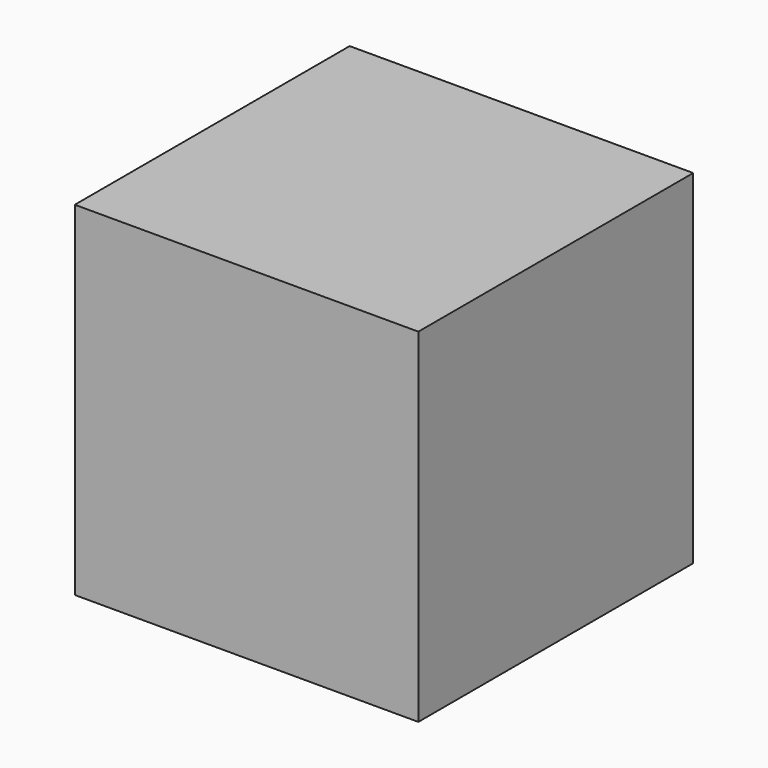
from build123d import *

# Parameters (mm, degrees)
F0_W     = 12.7
F0_H     = 12.7
F1_DEPTH = 12.7


# Not quite as in the source:
# - a length typed as a fraction of an inch, garbled in the dataset ("3 / 203.2 mm" for 3/8 in), is restored


with BuildPart() as f1:
    # F0 (on Top) → F1 (new body)
    with BuildSketch(Plane.XY):
        Rectangle(F0_W, F0_H)
    extrude(amount=F1_DEPTH)


solid = f1.part
